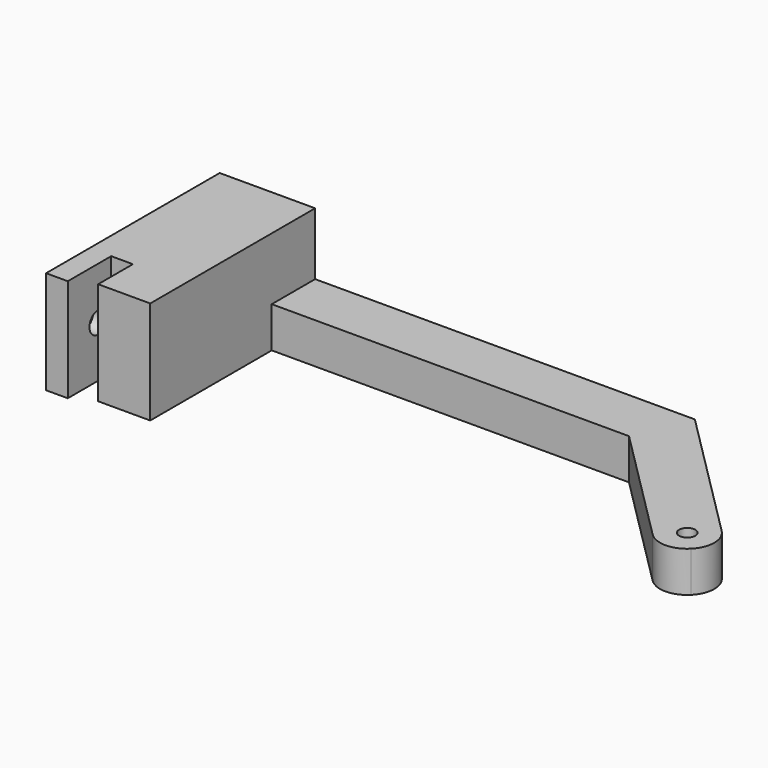
from build123d import *

# Parameters (mm, degrees)
F0_W      = 9.6
F0_H      = 19
F1_DEPTH  = 8
F2_W      = 4
F2_H      = 19
F2_W_2    = 9.6
F3_DEPTH  = 5
F4_W      = 4
F4_H      = 19
F5_DEPTH  = 10
F6_R      = 2
F7_DEPTH  = 4
F6_R_2    = 3.1
F8_DEPTH  = 1.5
F9_W      = 17.6
F9_H      = 7.5
F10_DEPTH = 25
F11_W     = 10
F11_H     = 7.5
F12_DEPTH = 70
F14_DEPTH = 25
F15_DEPTH = 40
F16_R     = 1.5
F17_DEPTH = 25
F18_DEPTH = 25
F20_DEPTH = 25
F21_R     = 4.99999


# Not quite as in the source:
# - a fillet or chamfer is up to 0.001 mm smaller than in the source, because OpenCascade refuses the exact size


with BuildPart() as f1:
    # F0 (on Front) → F1 (new body)
    with BuildSketch(Plane.XZ):
        Rectangle(F0_W, F0_H)
    extrude(amount=F1_DEPTH)

    # F2 (on face) → F3 (join)
    with BuildSketch(Plane(origin=(0, 0, 0), x_dir=(-1, 0, 0), z_dir=(0, 1, 0))):
        with Locations((6.8, 0)):
            Rectangle(F2_W, F2_H)
        Rectangle(F2_W_2, F2_H)
        with Locations((10.8, 0)):
            Rectangle(F2_W, F2_H)
    extrude(amount=F3_DEPTH)

    # F4 (on face) → F5 (join)
    with BuildSketch(Plane.XZ):
        with Locations((-10.8, 0)):
            Rectangle(F4_W, F4_H)
    extrude(amount=F5_DEPTH)

    # F6 (on face) → F7 (cut, through all)
    with BuildSketch(Plane(origin=(-12.8, 0, 0), x_dir=(0, -1, 0), z_dir=(-1, 0, 0))):
        with Locations((3, 0)):
            Circle(F6_R)
    extrude(amount=-F7_DEPTH, mode=Mode.SUBTRACT)

    # F6 (on face) → F8 (cut)
    with BuildSketch(Plane(origin=(-12.8, 0, 0), x_dir=(0, -1, 0), z_dir=(-1, 0, 0))):
        with Locations((3, 0)):
            Circle(F6_R_2)
        with Locations((3, 0)):
            Circle(F6_R, mode=Mode.SUBTRACT)
    extrude(amount=-F8_DEPTH, mode=Mode.SUBTRACT)

    # F9 (on face) → F10 (join)
    with BuildSketch(Plane(origin=(0, 5, 0), x_dir=(-1, 0, 0), z_dir=(0, 1, 0))):
        with Locations((4, -5.75)):
            Rectangle(F9_W, F9_H)
    extrude(amount=F10_DEPTH)

    # F11 (on face) → F12 (join)
    with BuildSketch(Plane.YZ.offset(4.8)):
        with Locations((25, -5.75)):
            Rectangle(F11_W, F11_H)
    extrude(amount=F12_DEPTH)

    # F13 (on face) → F14 (cut)
    with BuildSketch(Plane.XY.offset(-2)):
        Polygon((74.8, 30), (64.8, 20), (74.8, 20), align=None)
    extrude(amount=-F14_DEPTH, mode=Mode.SUBTRACT)

    # F15 (add): a face of the model
    f15_faces = [f1.faces().sort_by_distance(p)[0] for p in [
        (69.8, 25, -5.75),
    ]]
    extrude(f15_faces, amount=F15_DEPTH)

    # F16 (on face) → F17 (cut)
    with BuildSketch(Plane.XY.offset(-2)):
        with Locations((96.0132034356, 1.7157287525)):
            Circle(F16_R)
    extrude(amount=-F17_DEPTH, mode=Mode.SUBTRACT)

    # F18 (add): a face of the model
    f18_faces = [f1.faces().sort_by_distance(p)[0] for p in [
        (-4, 5, 3.75),
    ]]
    extrude(f18_faces, amount=F18_DEPTH)

    # F19 (on face) → F20 (cut)
    with BuildSketch(Plane.XY.offset(-2)):
        Polygon((93.0842712475, -8.2842712475), (96.0132034356, -5.3553390593), (70.6578643763, 20), (64.8, 20), align=None)
    extrude(amount=-F20_DEPTH, mode=Mode.SUBTRACT)

    # F21 (radius 5 in the source; OpenCascade refuses exactly that, so slightly less here)
    f21_edges = [f1.edges().sort_by_distance(p)[0] for p in [
        (96.013203, -5.355339, -5.75),
        (103.084271, 1.715729, -5.75),
    ]]
    fillet(f21_edges, radius=F21_R)


solid = f1.part
